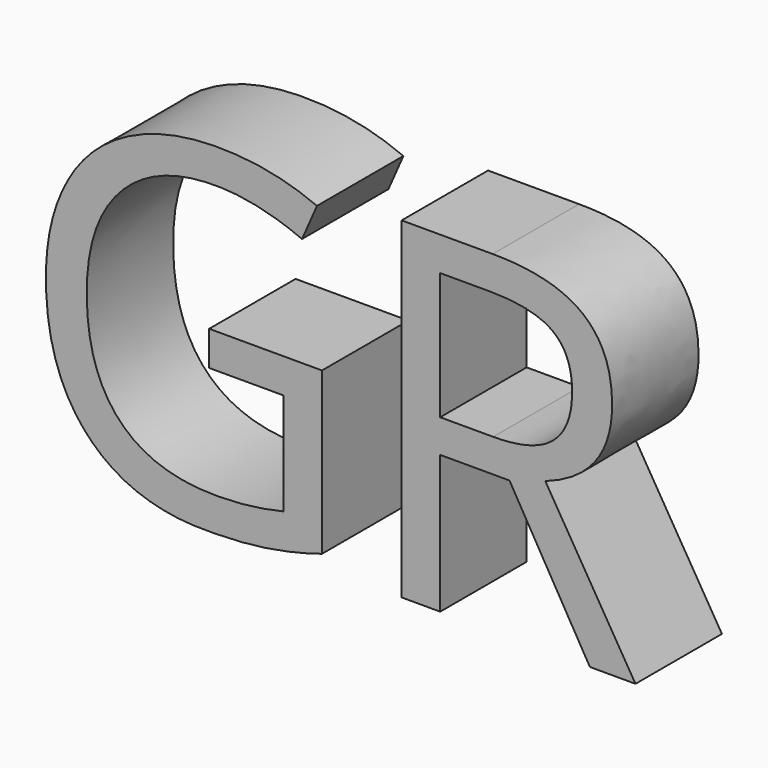
from build123d import *

# Parameters (mm, degrees)
F0_TEXT_SIZE = 54.6665172066
F1_DEPTH     = 12.7


# Not quite as in the source:
# - Text() gives the source's letters only with a copy of the font that has no kerning and outlines rounded to 1/6400 em; it was checked with that copy


with BuildPart() as f1:
    # F0 (on Front) → F1 (new body)
    with BuildSketch(Plane.XZ):
        with Locations((-32.1623034883, -21.7063805324)):
            Text('GR', F0_TEXT_SIZE, font='Open Sans', text_align=(TextAlign.LEFT, TextAlign.BOTTOM))
    extrude(amount=F1_DEPTH)


solid = f1.part
